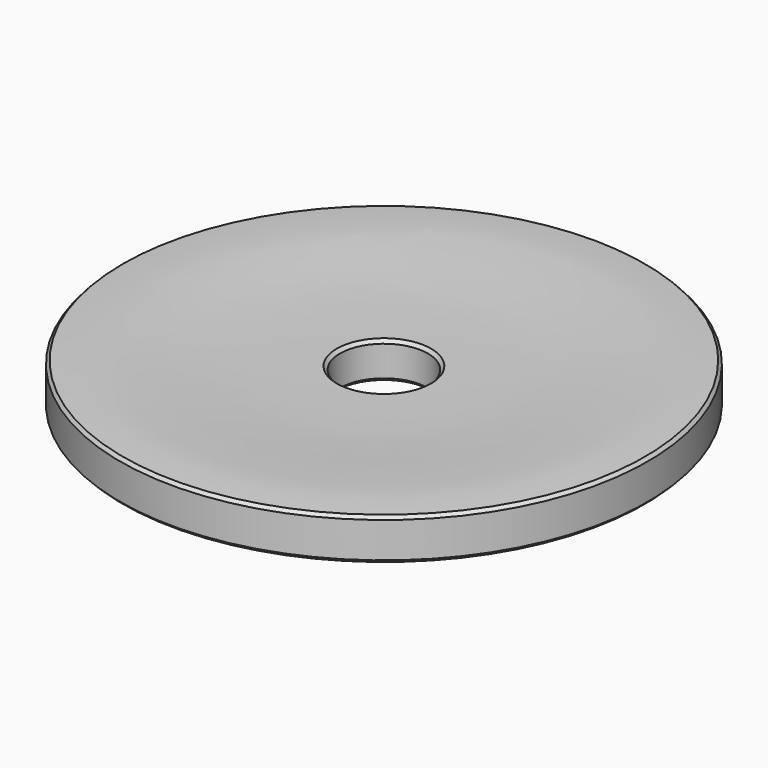
from build123d import *


# Not quite as in the source:
# - a fillet or chamfer that OpenCascade refuses, or shapes differently, is made with other operations: its cross-section is extruded or revolved along the edge and cut away or added


with BuildPart() as f1:
    # F0 (on Front) → F1 (revolve)
    with BuildSketch(Plane.XZ):
        with BuildLine():
            Line((-165, 0), (-27.5, 0))
            Line((-27.5, 0), (-27.5, 23))
            add(Edge.make_bspline(
                [(-165, 26), (-146.2488025427, 28), (-117.5518896036, 26.1885880856), (-84.9576765758, 23.5791079097), (-53.8473351003, 23.1516456126), (-37.6317065785, 23.0223040688), (-27.5, 23)],
                knots=[0, 0, 0, 0, 0.2991574258, 0.5427429345, 0.7774614784, 1, 1, 1, 1], degree=3))
            Line((-165, 26), (-165, 0))
        make_face()
    revolve(axis=Axis((0, 0, 18.2528793812), (0, 0, 1)))

    # F2: chamfer of 2 on 6 edges, made by hand

    # F2_s1 → F2_t2 (revolve, cut)
    with BuildSketch(Plane.XZ):
        with BuildLine():
            Line((-163.1402962248, 26.2435805193), (-165.0537542486, 24.1345180557))
            Line((-165.0537542486, 24.1345180557), (-165.0937542486, 24.1345180557))
            ThreePointArc((-165.0937542486, 24.1345180557), (-165.04, 25.0672590279), (-165.04, 26))
            Line((-165.04, 26), (-165.0042423314, 26.0397743966))
            ThreePointArc((-165.0042423314, 26.0397743966), (-164.0717010239, 26.1370271649), (-163.1441772343, 26.2833917961))
            Line((-163.1441772343, 26.2833917961), (-163.1402962248, 26.2435805193))
        make_face()
    revolve(axis=Axis((0, 0, 26), (0, 0, 1)), mode=Mode.SUBTRACT)

    # F2_s3 → F2_t4 (revolve, cut)
    with BuildSketch(Plane.XZ):
        with BuildLine():
            Line((-162.9434314575, -0.0565685425), (-165.0565685425, 2.0565685425))
            Line((-165.0565685425, 2.0565685425), (-165.0965685425, 2.0565685425))
            ThreePointArc((-165.0965685425, 2.0565685425), (-165.04, 1.0282842712), (-165.04, 0))
            Line((-165.04, 0), (-165, -0.04))
            ThreePointArc((-165, -0.04), (-163.9717157288, -0.04), (-162.9434314575, -0.0965685425))
            Line((-162.9434314575, -0.0965685425), (-162.9434314575, -0.0565685425))
        make_face()
    revolve(axis=Axis((0, 0, 0), (0, 0, 1)), mode=Mode.SUBTRACT)

    # F2_s5 → F2_t6 (revolve, cut)
    with BuildSketch(Plane.XZ):
        with BuildLine():
            Line((-29.5565685425, -0.0565685425), (-27.4434314575, 2.0565685425))
            Line((-27.4434314575, 2.0565685425), (-27.4034314575, 2.0565685425))
            ThreePointArc((-27.4034314575, 2.0565685425), (-27.46, 1.0282842712), (-27.46, 0))
            Line((-27.46, 0), (-27.5, -0.04))
            ThreePointArc((-27.5, -0.04), (-28.5282842712, -0.04), (-29.5565685425, -0.0965685425))
            Line((-29.5565685425, -0.0965685425), (-29.5565685425, -0.0565685425))
        make_face()
    revolve(axis=Axis((0, 0, 0), (0, 0, 1)), mode=Mode.SUBTRACT)

    # F2_s7 → F2_t8 (revolve, cut)
    with BuildSketch(Plane.XZ):
        with BuildLine():
            Line((-27.4435110484, 20.9483524934), (-29.5508649872, 23.0616406292))
            Line((-29.5508649872, 23.0616406292), (-29.5507525079, 23.1016404711))
            ThreePointArc((-29.5507525079, 23.1016404711), (-28.5254033873, 23.0424149132), (-27.4999119437, 23.0399999031))
            Line((-27.4999119437, 23.0399999031), (-27.46, 23))
            ThreePointArc((-27.46, 23), (-27.46, 21.9741762467), (-27.4035110484, 20.9483524934))
            Line((-27.4035110484, 20.9483524934), (-27.4435110484, 20.9483524934))
        make_face()
    revolve(axis=Axis((0, 0, 23), (0, 0, 1)), mode=Mode.SUBTRACT)


solid = f1.part
